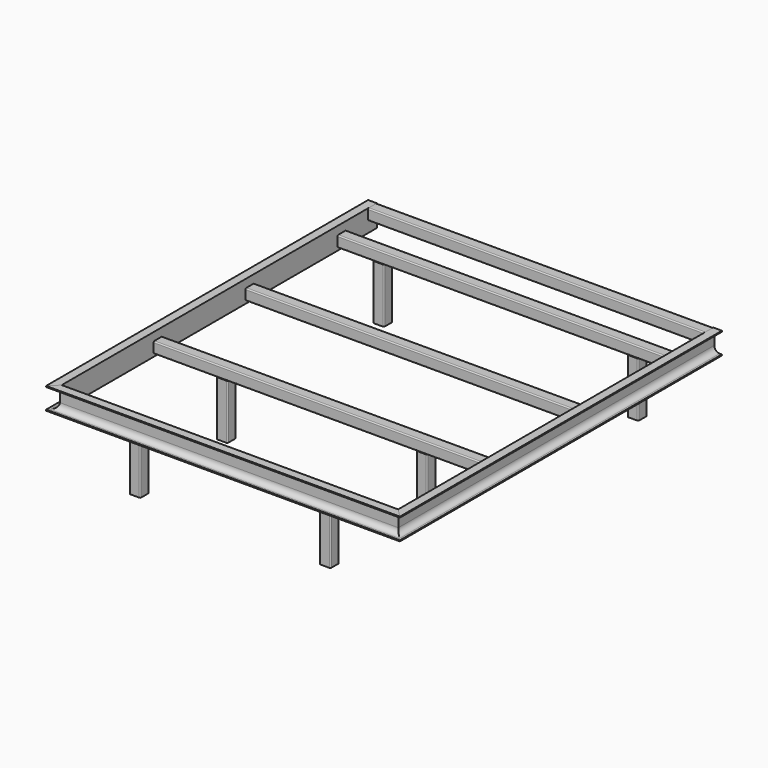
from build123d import *

# Parameters (mm, degrees)
F0_W           = 50.8
F0_H           = 50.8
F0_W_2         = 38.1
F0_H_2         = 38.1
F1_DEPTH       = 254
F2_W           = 50.8
F2_H           = 50.8
F2_W_2         = 38.1
F2_H_2         = 38.1
F3_DEPTH       = 781.05
F4_W           = 50.8
F4_H           = 50.8
F4_W_2         = 38.1
F4_H_2         = 38.1
F5_DEPTH       = 781.05
F6_W           = 50.8
F6_H           = 50.8
F6_W_2         = 38.1
F6_H_2         = 38.1
F7_DEPTH       = 781.05
F9_DEPTH       = 1665.8336
F9_DEPTH_BACK  = 203.2
F10_R          = 25.4
F12_R          = 5.08
F12_2_R        = 5.08
F12_3_R        = 5.08
F12_4_R        = 5.08
F12_5_R        = 5.08
F12_6_R        = 5.08
F12_7_R        = 5.08
F12_8_R        = 5.08
F12_9_R        = 5.08
F14_DEPTH      = 821.2836
F15_R          = 25.4
F16_T1_DEPTH   = 308.5361293293
F17_T1_DEPTH   = 308.5361293293
F18_T1_DEPTH   = 308.5361293293
F18_2_T1_DEPTH = 308.5361293293
F19_W          = 50.8
F19_H          = 50.8
F19_W_2        = 38.1
F19_H_2        = 38.1
F20_DEPTH      = 781.05
F21_R          = 5.08
F22_W          = 50.8
F22_H          = 50.8
F22_W_2        = 38.1
F22_H_2        = 38.1
F23_DEPTH      = 781.05
F24_R          = 5.08


# Not quite as in the source:
# - a fillet or chamfer that OpenCascade refuses, or shapes differently, is made with other operations: its cross-section is extruded or revolved along the edge and cut away or added


with BuildPart() as f1:
    # F0 (on Top) → F1 (new body)
    with BuildSketch(Plane.XY):
        with Locations((-590.55, 0)):
            Rectangle(F0_W, F0_H)
        with Locations((-590.55, 0)):
            Rectangle(F0_W_2, F0_H_2, mode=Mode.SUBTRACT)
    extrude(amount=F1_DEPTH)

    # F12#7
    f12_7_edges = [f1.edges().sort_by_distance(p)[0] for p in [
        (-615.95, 25.4, 127),
        (-615.95, -25.4, 127),
        (-565.15, 25.4, 127),
        (-565.15, -25.4, 127),
    ]]
    fillet(f12_7_edges, radius=F12_7_R)


with BuildPart() as f1b:
    # F0 (on Top) → F1, piece 2 (new body)
    with BuildSketch(Plane.XY):
        with Locations((-463.55, -1066.8)):
            Rectangle(F0_W, F0_H)
        with Locations((-463.55, -1066.8)):
            Rectangle(F0_W_2, F0_H_2, mode=Mode.SUBTRACT)
    extrude(amount=F1_DEPTH)

    # F12#6
    f12_6_edges = [f1b.edges().sort_by_distance(p)[0] for p in [
        (-438.15, -1041.4, 127),
        (-438.15, -1092.2, 127),
        (-488.95, -1092.2, 127),
        (-488.95, -1041.4, 127),
    ]]
    fillet(f12_6_edges, radius=F12_6_R)


with BuildPart() as f1c:
    # F0 (on Top) → F1, piece 3 (new body)
    with BuildSketch(Plane.XY):
        with Locations((-441.325, -1600.2)):
            Rectangle(F0_W, F0_H)
        with Locations((-441.325, -1600.2)):
            Rectangle(F0_W_2, F0_H_2, mode=Mode.SUBTRACT)
    extrude(amount=F1_DEPTH)

    # F12#2
    f12_2_edges = [f1c.edges().sort_by_distance(p)[0] for p in [
        (-415.925, -1625.6, 127),
        (-466.725, -1625.6, 127),
        (-466.725, -1574.8, 127),
        (-415.925, -1574.8, 127),
    ]]
    fillet(f12_2_edges, radius=F12_2_R)


with BuildPart() as f1d:
    # F0 (on Top) → F1, piece 4 (new body)
    with BuildSketch(Plane.XY):
        with Locations((590.55, 0)):
            Rectangle(F0_W, F0_H)
        with Locations((590.55, 0)):
            Rectangle(F0_W_2, F0_H_2, mode=Mode.SUBTRACT)
    extrude(amount=F1_DEPTH)

    # F12#9
    f12_9_edges = [f1d.edges().sort_by_distance(p)[0] for p in [
        (615.95, 25.4, 127),
        (565.15, 25.4, 127),
        (565.15, -25.4, 127),
        (615.95, -25.4, 127),
    ]]
    fillet(f12_9_edges, radius=F12_9_R)


with BuildPart() as f1e:
    # F0 (on Top) → F1, piece 5 (new body)
    with BuildSketch(Plane.XY):
        with Locations((441.325, -1600.2)):
            Rectangle(F0_W, F0_H)
        with Locations((441.325, -1600.2)):
            Rectangle(F0_W_2, F0_H_2, mode=Mode.SUBTRACT)
    extrude(amount=F1_DEPTH)

    # F12#3
    f12_3_edges = [f1e.edges().sort_by_distance(p)[0] for p in [
        (415.925, -1625.6, 127),
        (466.725, -1625.6, 127),
        (415.925, -1574.8, 127),
        (466.725, -1574.8, 127),
    ]]
    fillet(f12_3_edges, radius=F12_3_R)


with BuildPart() as f1f:
    # F0 (on Top) → F1, piece 6 (new body)
    with BuildSketch(Plane.XY):
        with Locations((463.55, -1066.8)):
            Rectangle(F0_W, F0_H)
        with Locations((463.55, -1066.8)):
            Rectangle(F0_W_2, F0_H_2, mode=Mode.SUBTRACT)
    extrude(amount=F1_DEPTH)

    # F12#5
    f12_5_edges = [f1f.edges().sort_by_distance(p)[0] for p in [
        (488.95, -1092.2, 127),
        (438.15, -1092.2, 127),
        (488.95, -1041.4, 127),
        (438.15, -1041.4, 127),
    ]]
    fillet(f12_5_edges, radius=F12_5_R)


with BuildPart() as f3:
    # F2 (on Right) → F3 (new body, symmetric)
    with BuildSketch(Plane.YZ):
        with Locations((0, 279.4)):
            Rectangle(F2_W, F2_H)
        with Locations((0, 279.4)):
            Rectangle(F2_W_2, F2_H_2, mode=Mode.SUBTRACT)
    extrude(amount=F3_DEPTH, both=True)

    # F12#8
    f12_8_edges = [f3.edges().sort_by_distance(p)[0] for p in [
        (0, -25.4, 254),
        (0, 25.4, 254),
        (0, 25.4, 304.8),
        (0, -25.4, 304.8),
    ]]
    fillet(f12_8_edges, radius=F12_8_R)


with BuildPart() as f5:
    # F4 (on Right) → F5 (new body, symmetric)
    with BuildSketch(Plane.YZ):
        with Locations((-1066.8, 279.4)):
            Rectangle(F4_W, F4_H)
        with Locations((-1066.8, 279.4)):
            Rectangle(F4_W_2, F4_H_2, mode=Mode.SUBTRACT)
    extrude(amount=F5_DEPTH, both=True)

    # F12#4
    f12_4_edges = [f5.edges().sort_by_distance(p)[0] for p in [
        (0, -1092.2, 254),
        (0, -1041.4, 254),
        (0, -1041.4, 304.8),
        (0, -1092.2, 304.8),
    ]]
    fillet(f12_4_edges, radius=F12_4_R)


with BuildPart() as f7:
    # F6 (on Right) → F7 (new body, symmetric)
    with BuildSketch(Plane.YZ):
        with Locations((-1600.2, 279.4)):
            Rectangle(F6_W, F6_H)
        with Locations((-1600.2, 279.4)):
            Rectangle(F6_W_2, F6_H_2, mode=Mode.SUBTRACT)
    extrude(amount=F7_DEPTH, both=True)

    # F12
    f12_edges = [f7.edges().sort_by_distance(p)[0] for p in [
        (0, -1625.6, 304.8),
        (0, -1625.6, 254),
        (0, -1574.8, 304.8),
        (0, -1574.8, 254),
    ]]
    fillet(f12_edges, radius=F12_R)


with BuildPart() as f9:
    # F8 (on Front) → F9 (new body, two sides)
    with BuildSketch(Plane.XZ) as f9_sk:
        Polygon((-781.05, 342.9), (-821.2836, 342.9), (-821.2836, 338.2264), (-785.7236, 338.2264), (-785.7236, 245.9736), (-821.2836, 245.9736), (-821.2836, 241.3), (-781.05, 241.3), align=None)
    extrude(amount=F9_DEPTH)
    extrude(f9_sk.sketch, amount=-F9_DEPTH_BACK)

    # F10
    f10_edges = [f9.edges().sort_by_distance(p)[0] for p in [
        (-785.7236, -731.3168, 338.2264),
        (-785.7236, -731.3168, 245.9736),
    ]]
    fillet(f10_edges, radius=F10_R)


with BuildPart() as f11_1:
    # F11: instance of F9
    add(f9.part.mirror(Plane.YZ))

    # F18: chamfer of 40.2336 on 1 edges, made by hand

    # F18_s2 → F18_t1 (cut)
    with BuildSketch(Plane.XY.offset(137.8319353354)):
        Polygon((781.05, -1625.6), (821.2836, -1665.8336), (781.05, -1665.8336), align=None)
    extrude(amount=F18_T1_DEPTH, mode=Mode.SUBTRACT)


with BuildPart() as f14:
    # F13 (on Right) → F14 (new body, symmetric)
    with BuildSketch(Plane.YZ):
        Polygon((-1625.6, 342.9), (-1665.8336, 342.9), (-1665.8336, 338.2264), (-1630.2736, 338.2264), (-1630.2736, 245.9736), (-1665.8336, 245.9736), (-1665.8336, 241.3), (-1625.6, 241.3), align=None)
    extrude(amount=F14_DEPTH, both=True)

    # F15
    f15_edges = [f14.edges().sort_by_distance(p)[0] for p in [
        (0, -1630.2736, 245.9736),
        (0, -1630.2736, 338.2264),
    ]]
    fillet(f15_edges, radius=F15_R)

    # F16: chamfer of 40.2336 on 1 edges, made by hand

    # F16_s2 → F16_t1 (cut)
    with BuildSketch(Plane.XY.offset(137.8319353354)):
        Polygon((-821.2836, -1665.8336), (-781.05, -1625.6), (-821.2836, -1625.6), align=None)
    extrude(amount=F16_T1_DEPTH, mode=Mode.SUBTRACT)

    # F18#2: chamfer of 40.2336 on 1 edges, made by hand

    # F18_2_s2 → F18_2_t1 (cut)
    with BuildSketch(Plane.XY.offset(137.8319353354)):
        Polygon((821.2836, -1665.8336), (781.05, -1625.6), (821.2836, -1625.6), align=None)
    extrude(amount=F18_2_T1_DEPTH, mode=Mode.SUBTRACT)


with BuildPart() as f9_1:
    add(f9.part)

    # F17: chamfer of 40.2336 on 1 edges, made by hand

    # F17_s2 → F17_t1 (cut)
    with BuildSketch(Plane.XY.offset(137.8319353354)):
        Polygon((-781.05, -1625.6), (-821.2836, -1665.8336), (-781.05, -1665.8336), align=None)
    extrude(amount=F17_T1_DEPTH, mode=Mode.SUBTRACT)


with BuildPart() as f20:
    # F19 (on Right) → F20 (new body, symmetric)
    with BuildSketch(Plane.YZ):
        with Locations((177.8, 317.5)):
            Rectangle(F19_W, F19_H)
        with Locations((177.8, 317.5)):
            Rectangle(F19_W_2, F19_H_2, mode=Mode.SUBTRACT)
    extrude(amount=F20_DEPTH, both=True)

    # F21
    f21_edges = [f20.edges().sort_by_distance(p)[0] for p in [
        (0, 152.4, 342.9),
        (0, 152.4, 292.1),
        (0, 203.2, 342.9),
        (0, 203.2, 292.1),
    ]]
    fillet(f21_edges, radius=F21_R)


with BuildPart() as f23:
    # F22 (on Right) → F23 (new body, symmetric)
    with BuildSketch(Plane.YZ):
        with Locations((-533.4, 279.4)):
            Rectangle(F22_W, F22_H)
        with Locations((-533.4, 279.4)):
            Rectangle(F22_W_2, F22_H_2, mode=Mode.SUBTRACT)
    extrude(amount=F23_DEPTH, both=True)

    # F24
    f24_edges = [f23.edges().sort_by_distance(p)[0] for p in [
        (0, -508, 304.8),
        (0, -508, 254),
        (0, -558.8, 304.8),
        (0, -558.8, 254),
    ]]
    fillet(f24_edges, radius=F24_R)


solid = Compound([f1.part, f1b.part, f1c.part, f1d.part, f1e.part, f1f.part, f3.part, f5.part, f7.part, f11_1.part, f14.part, f9_1.part, f20.part, f23.part])
